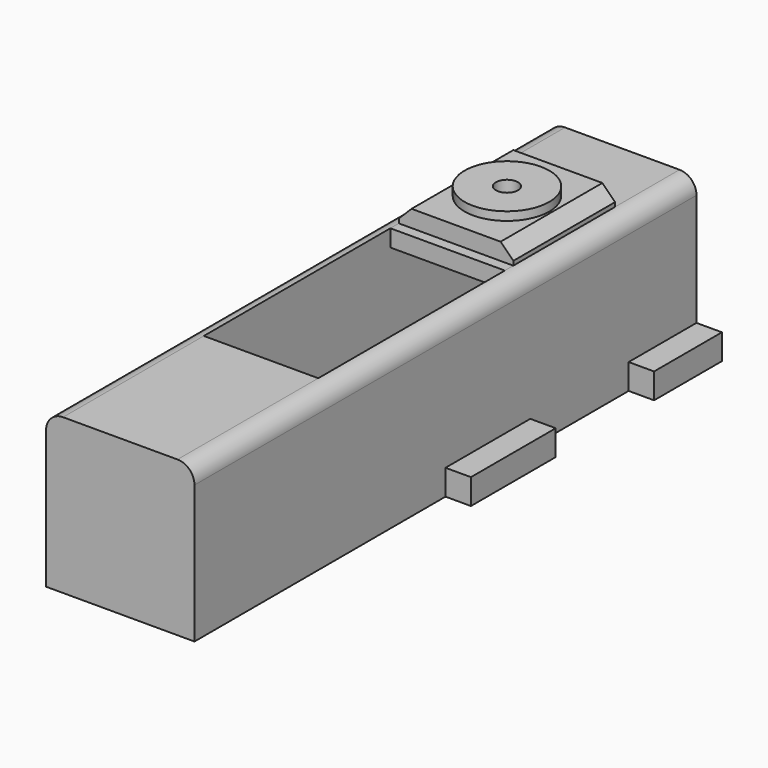
from build123d import *

# Parameters (mm, degrees)
F0_W          = 44.45
F0_H          = 187.96
F1_DEPTH      = 46.355
F2_R          = 5.08
F3_W          = 34.29
F3_H          = 38.1
F4_DEPTH      = 5.08
F5_R          = 12.7
F6_DEPTH      = 2.54
F7_W          = 31.75
F7_H          = 7.62
F8_DEPTH      = 7.62
F9_W          = 31.75
F9_H          = 7.62
F10_DEPTH     = 7.62
F11_W         = 25.4
F11_H         = 7.62
F12_DEPTH     = 7.62
F13_W         = 25.4
F13_H         = 7.62
F14_DEPTH     = 7.62
F15_SIZE      = 3.81
F16_T         = 5.08
F16_T3_DEPTH  = 44.45
F16_T5_DEPTH  = 48.26
F16_T7_DEPTH  = 35.56
F16_T9_DEPTH  = 17.78
F16_T11_DEPTH = 41.91
F17_W         = 34.29
F17_H         = 69.85
F18_DEPTH     = 25.4
F19_R         = 3.302
F20_DEPTH     = 53.976


# Not quite as in the source:
# - a shell that OpenCascade refuses in one call is made with other operations: the cavity is built on its own and cut out


with BuildPart() as f1:
    # F0 (on Top) → F1 (new body)
    with BuildSketch(Plane.XY):
        Rectangle(F0_W, F0_H)
    extrude(amount=F1_DEPTH)

    # F2
    f2_edges = [f1.edges().sort_by_distance(p)[0] for p in [
        (22.225, 0, 46.355),
        (-22.225, 0, 46.355),
    ]]
    fillet(f2_edges, radius=F2_R)

    # F3 (on face) → F4 (join)
    with BuildSketch(Plane.XY.offset(46.355)):
        with Locations((0, 50.8)):
            Rectangle(F3_W, F3_H)
    extrude(amount=F4_DEPTH)

    # F5 (on face) → F6 (join)
    with BuildSketch(Plane.XY.offset(51.435)):
        with Locations((0, 50.8)):
            Circle(F5_R)
    extrude(amount=F6_DEPTH)

    # F7 (on face) → F8 (join)
    with BuildSketch(Plane.YZ.offset(22.225)):
        with Locations((15.875, 3.81)):
            Rectangle(F7_W, F7_H)
    extrude(amount=F8_DEPTH)

    # F9 (on face) → F10 (join)
    with BuildSketch(Plane(origin=(-22.225, 0, 0), x_dir=(0, -1, 0), z_dir=(-1, 0, 0))):
        with Locations((-15.875, 3.81)):
            Rectangle(F9_W, F9_H)
    extrude(amount=F10_DEPTH)

    # F11 (on face) → F12 (join)
    with BuildSketch(Plane(origin=(-22.225, 0, 0), x_dir=(0, -1, 0), z_dir=(-1, 0, 0))):
        with Locations((-81.28, 3.81)):
            Rectangle(F11_W, F11_H)
    extrude(amount=F12_DEPTH)

    # F13 (on face) → F14 (join)
    with BuildSketch(Plane.YZ.offset(22.225)):
        with Locations((81.28, 3.81)):
            Rectangle(F13_W, F13_H)
    extrude(amount=F14_DEPTH)

    # F15
    f15_edges = [f1.edges().sort_by_distance(p)[0] for p in [
        (-17.145, 50.8, 51.435),
        (17.145, 50.8, 51.435),
    ]]
    chamfer(f15_edges, length=F15_SIZE)

    # F16: shell of thickness 5.08, made by hand


with BuildPart() as f16_core1:
    # F16_t2: copy of F1
    add(f1.part)

    # the walls: a layer under each face that stays
    f16_faces = [f16_core1.faces().sort_by_distance(p)[0] for p in [
        (0, 31.75, 48.895),
        (-17.145, 50.8, 46.99),
        (-15.24, 50.8, 49.53),
        (0, -31.115, 46.355),
        (-8.89, 38.1, 51.435),
        (17.145, 50.8, 46.99),
        (15.24, 50.8, 49.53),
        (0, 69.85, 48.895),
        (0, -93.98, 23.1775),
        (-12.7, 50.8, 52.705),
        (0, 81.915, 46.355),
        (0, 93.98, 23.1775),
        (-22.225, 0, 20.6375),
        (22.225, 0, 20.6375),
        (0, 50.8, 53.975),
        (-26.035, 81.28, 7.62),
        (-29.845, 81.28, 3.81),
        (29.845, 81.28, 3.81),
        (26.035, 81.28, 7.62),
        (-26.035, 68.58, 3.81),
        (-26.035, 31.75, 3.81),
        (-26.035, 15.875, 7.62),
        (-26.035, 0, 3.81),
        (26.035, 0, 3.81),
        (26.035, 15.875, 7.62),
        (26.035, 31.75, 3.81),
        (26.035, 68.58, 3.81),
        (-29.845, 15.875, 3.81),
        (29.845, 15.875, 3.81),
    ]]
    thicken(f16_faces, amount=-F16_T, mode=Mode.SUBTRACT)

    # F16_s4 → F16_t3 (cut)
    with BuildSketch(Plane.YZ.offset(-22.225)):
        Polygon((31.6992, 46.4058), (36.83, 46.355), (36.83, 41.275), (31.75, 41.275), align=None)
        Polygon((69.9008, 46.4058), (64.77, 46.355), (64.77, 41.275), (69.85, 41.275), align=None)
    extrude(amount=F16_T3_DEPTH, mode=Mode.SUBTRACT)

    # F16_s6 → F16_t5 (cut)
    with BuildSketch(Plane.XZ.offset(-74.93)):
        Polygon((-17.1958, 46.4058), (-12.065, 46.355), (-12.065, 41.275), (-17.145, 41.275), align=None)
        Polygon((17.1958, 46.4058), (12.065, 46.355), (12.065, 41.275), (17.145, 41.275), align=None)
    extrude(amount=F16_T5_DEPTH, mode=Mode.SUBTRACT)

    # F16_s8 → F16_t7 (cut)
    with BuildSketch(Plane.XZ.offset(-99.06)):
        Polygon((-22.2758, 7.6708), (-17.145, 7.62), (-17.145, 2.54), (-22.225, 2.54), align=None)
        Polygon((22.2758, 7.6708), (17.145, 7.62), (17.145, 2.54), (22.225, 2.54), align=None)
    extrude(amount=F16_T7_DEPTH, mode=Mode.SUBTRACT)

    # F16_s10 → F16_t9 (cut)
    with BuildSketch(Plane.XY.offset(-5.08)):
        Polygon((-22.2758, 68.5292), (-17.145, 68.58), (-17.145, 73.66), (-22.225, 73.66), align=None)
        Polygon((-22.2758, 31.8008), (-17.145, 31.75), (-17.145, 26.67), (-22.225, 26.67), align=None)
        Polygon((-22.2758, -0.0508), (-17.145, 0), (-17.145, 5.08), (-22.225, 5.08), align=None)
        Polygon((22.2758, -0.0508), (17.145, 0), (17.145, 5.08), (22.225, 5.08), align=None)
        Polygon((22.2758, 31.8008), (17.145, 31.75), (17.145, 26.67), (22.225, 26.67), align=None)
        Polygon((22.2758, 68.5292), (17.145, 68.58), (17.145, 73.66), (22.225, 73.66), align=None)
    extrude(amount=F16_T9_DEPTH, mode=Mode.SUBTRACT)

    # F16_s12 → F16_t11 (cut)
    with BuildSketch(Plane.XZ.offset(-36.83)):
        Polygon((-22.2758, 7.6708), (-17.145, 7.62), (-17.145, 2.54), (-22.225, 2.54), align=None)
        Polygon((22.2758, 7.6708), (17.145, 7.62), (17.145, 2.54), (22.225, 2.54), align=None)
    extrude(amount=F16_T11_DEPTH, mode=Mode.SUBTRACT)

    # F16_s13 → F16_t14 (revolve, cut)
    with BuildSketch(Plane.XZ.offset(-50.8)):
        Polygon((12.7508, 51.4858), (12.7, 46.355), (7.62, 46.355), (7.62, 51.435), align=None)
    revolve(axis=Axis((0, 50.8, 51.435), (0, 0, 1)), mode=Mode.SUBTRACT)


with BuildPart() as f1_1:
    add(f1.part)

    # what is left inside the walls is the cavity
    f16_cavity = [f16_core1.part.solids().sort_by_distance(p)[0] for p in [
        (17.0942, 0, 27.516667),
    ]]
    add(f16_cavity, mode=Mode.SUBTRACT)

    # F17 (on face) → F18 (cut)
    with BuildSketch(Plane.XY.offset(46.355)):
        with Locations((0, -6.35)):
            Rectangle(F17_W, F17_H)
    extrude(amount=-F18_DEPTH, mode=Mode.SUBTRACT)

    # F19 (on face) → F20 (cut, through all)
    with BuildSketch(Plane.XY.offset(53.975)):
        with Locations((0, 50.8)):
            Circle(F19_R)
    extrude(amount=-F20_DEPTH, mode=Mode.SUBTRACT)


solid = f1_1.part
